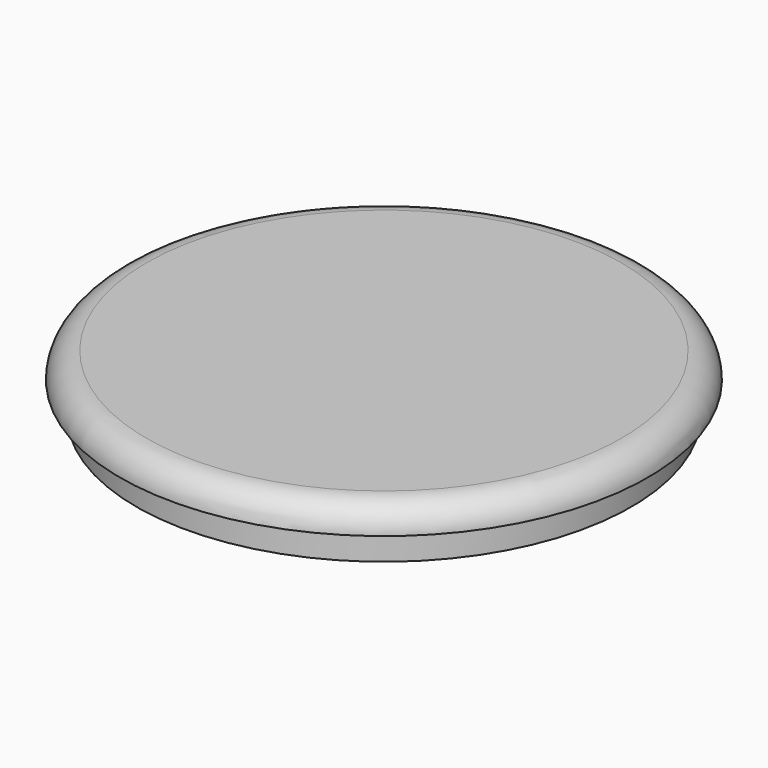
from build123d import *


# Not quite as in the source:
# - a fillet or chamfer that OpenCascade refuses, or shapes differently, is made with other operations: its cross-section is extruded or revolved along the edge and cut away or added


with BuildPart() as f1:
    # F0 (on Front) → F1 (revolve)
    with BuildSketch(Plane.XZ):
        Polygon((-9.525, 0), (0, 0), (0, 2.2), (-10.16, 2.2), (-10.16, 1.2), (-9.525, 1.2), align=None)
    revolve(axis=Axis((0, 0, 1.1), (0, 0, -1)))

    # F2: fillet of radius 1.016 on 1 edges, made by hand

    # F2_s1 → F2_t2 (revolve, cut)
    with BuildSketch(Plane.XZ):
        with BuildLine():
            ThreePointArc((-9.144, 2.2), (-9.8624204897, 1.9024204897), (-10.16, 1.184))
            Line((-10.16, 1.184), (-10.16, 2.2))
            Line((-10.16, 2.2), (-9.144, 2.2))
        make_face()
    revolve(axis=Axis((0, 0, 2.2), (0, 0, -1)), mode=Mode.SUBTRACT)


solid = f1.part
